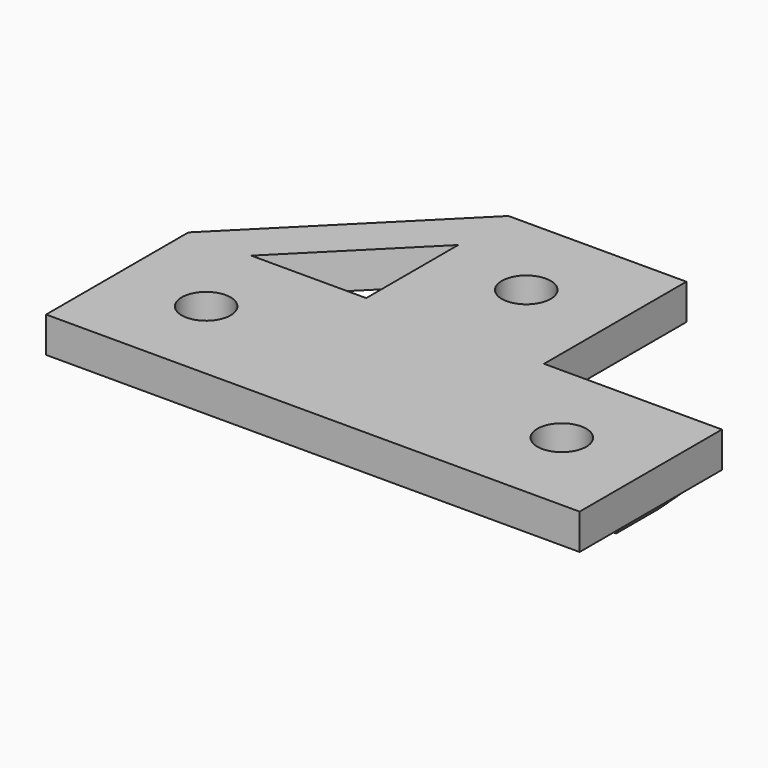
from build123d import *

# Parameters (mm, degrees)
F1_DEPTH = 4
F3_DEPTH = 60
F5_DEPTH = 20
F6_SIZE  = 1.49999
F7_R     = 2.75
F8_DEPTH = 5.501


# Not quite as in the source:
# - a fillet or chamfer is up to 0.001 mm smaller than in the source, because OpenCascade refuses the exact size


with BuildPart() as f1:
    # F0 (on Top) → F1 (new body)
    with BuildSketch(Plane.XY):
        Polygon((0, 20), (0, 0), (60, 0), (60, 20), (40, 20), (40, 40), (20, 40), align=None)
        Polygon((20, 32.9289321881), (20, 20), (7.0710678119, 20), align=None, mode=Mode.SUBTRACT)
    extrude(amount=F1_DEPTH)

    # F2 (on face) → F3 (join, through all)
    with BuildSketch(Plane.YZ.offset(60)):
        Polygon((14.5, 0), (5.5, 0), (7, -1.5), (13, -1.5), align=None)
    extrude(amount=-F3_DEPTH)

    # F4 (on face) → F5 (join, through all)
    with BuildSketch(Plane(origin=(0, 40, 0), x_dir=(-1, 0, 0), z_dir=(0, 1, 0))):
        Polygon((-25.5, 0), (-34.5, 0), (-33, -1.5), (-27, -1.5), align=None)
    extrude(amount=-F5_DEPTH)

    # F6 (size 1.5 in the source; OpenCascade refuses exactly that, so slightly less here)
    f6_edges = [f1.edges().sort_by_distance(p)[0] for p in [
        (60, 10, -1.5),
        (0, 10, -1.5),
        (30, 20, -1.5),
        (30, 40, -1.5),
    ]]
    chamfer(f6_edges, length=F6_SIZE)

    # F7 (on face) → F8 (cut, through all)
    with BuildSketch(Plane.XY.offset(4)):
        with Locations((30, 30)):
            Circle(F7_R)
        with Locations((10, 10)):
            Circle(F7_R)
        with Locations((50, 10)):
            Circle(F7_R)
    extrude(amount=-F8_DEPTH, mode=Mode.SUBTRACT)


solid = f1.part
